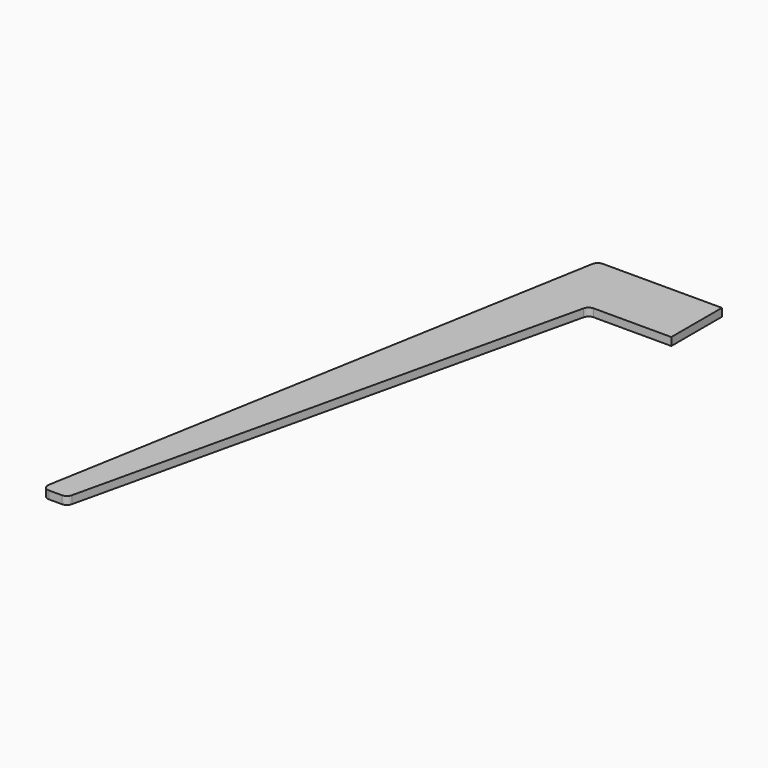
from build123d import *

# Parameters (mm, degrees)
F1_DEPTH = 15.875
F2_R     = 12.7


# Not quite as in the source:
# - a length typed as a fraction of an inch, garbled in the dataset ("3 / 203.2 mm" for 3/8 in), is restored


with BuildPart() as f1:
    # F0 (on Top) → F1 (new body)
    with BuildSketch(Plane.XY):
        Polygon((201.5417389498, 1143), (0, 0), (50.8, 0), (285.3620821836, 1016), (451.3084056164, 1016), (451.3084056164, 1143), align=None)
    extrude(amount=F1_DEPTH)

    # F2
    f2_edges = [f1.edges().sort_by_distance(p)[0] for p in [
        (201.541739, 1143, 7.9375),
        (285.362082, 1016, 7.9375),
        (0, 0, 7.9375),
        (50.8, 0, 7.9375),
    ]]
    fillet(f2_edges, radius=F2_R)


solid = f1.part
